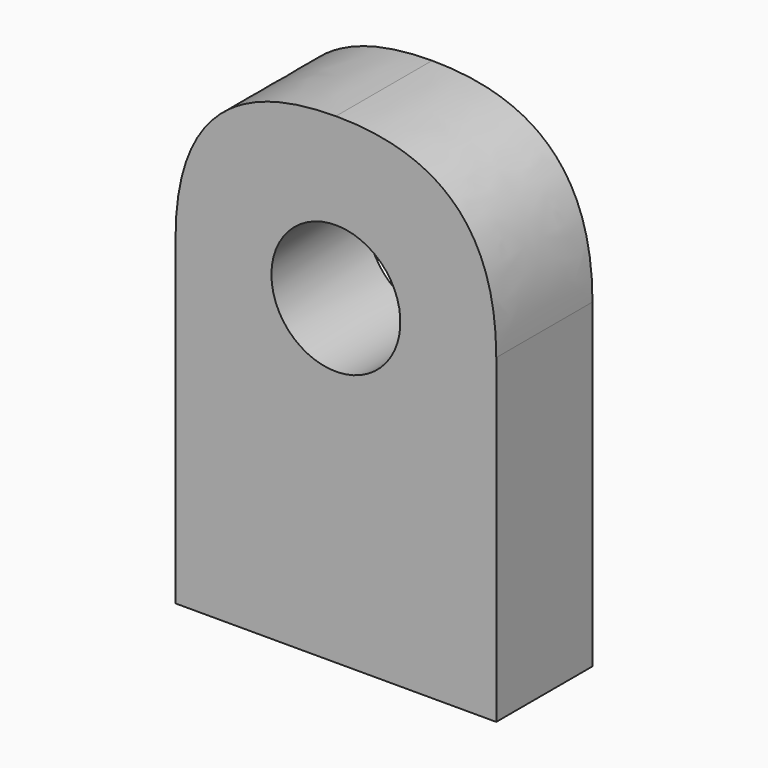
from build123d import *

# Parameters (mm, degrees)
F0_W        = 4.7625
F0_H        = 19.05
F1_DEPTH    = 12.7
F3_T1_DEPTH = 36.5125
F4_D        = 5.1054


# Not quite as in the source:
# - a fillet or chamfer that OpenCascade refuses, or shapes differently, is made with other operations: its cross-section is extruded or revolved along the edge and cut away or added


with BuildPart() as f1:
    # F0 (on Right) → F1 (new body)
    with BuildSketch(Plane.YZ):
        with Locations((2.38125, -9.525)):
            Rectangle(F0_W, F0_H)
    extrude(amount=F1_DEPTH)

    # F3: fillet of radius 6.35 on 2 edges, made by hand

    # F3_s2 → F3_t1 (cut)
    with BuildSketch(Plane.XZ.offset(-20.6375)):
        with BuildLine():
            add(Edge.make_bspline(
                [(6.35, 0), (0, 0), (0, -6.35)],
                knots=[0, 0, 0, 1, 1, 1], degree=2, weights=[1, 1, 1]))
            Line((0, -6.35), (0, 0))
            Line((0, 0), (6.35, 0))
        make_face()
        with BuildLine():
            add(Edge.make_bspline(
                [(6.35, 0), (12.7, 0), (12.7, -6.35)],
                knots=[0, 0, 0, 1, 1, 1], degree=2, weights=[1, 1, 1]))
            Line((12.7, -6.35), (12.7, 0))
            Line((12.7, 0), (6.35, 0))
        make_face()
    extrude(amount=F3_T1_DEPTH, mode=Mode.SUBTRACT)

    # F4 (through all)
    with Locations(Plane.XZ):
        with Locations((6.35, -6.35)):
            Hole(F4_D / 2)


solid = f1.part
